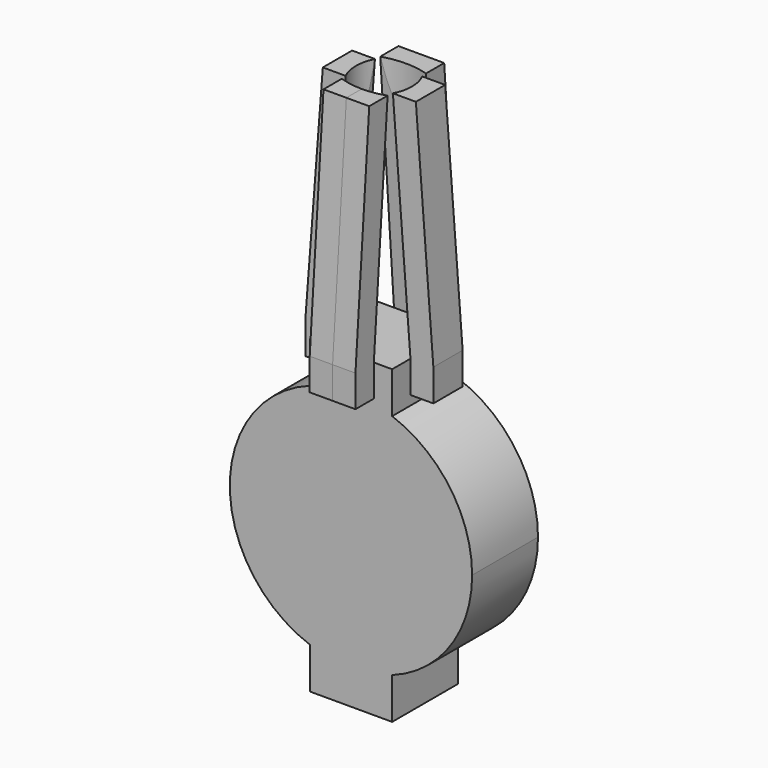
from build123d import *

# Parameters (mm, degrees)
F0_W      = 4.565686686
F0_H      = 1.0178177617
F0_H_2    = 1.0234280489
F0_H_3    = 0.7616141811
F0_H_4    = 0.7546050474
F1_DEPTH  = 4.572
F3_DEPTH  = 1.27
F4_DEPTH  = 1.27
F6_DEPTH  = 3.302
F8_DEPTH  = 1.27
F10_DEPTH = 10.16
F12_DEPTH = 10.16
F14_DEPTH = 10.16
F16_DEPTH = 10.16


with BuildPart() as f1:
    # F0 (on Front) → F1 (new body)
    with BuildSketch(Plane.XZ):
        with BuildLine():
            ThreePointArc((2.2870195098, -6.3278463876), (5.5072772106, -3.865487792), (6.7284543651, 0))
            ThreePointArc((6.7284543651, 0), (5.5072772106, 3.865487792), (2.2870195098, 6.3278463876))
            Line((2.2870195098, 6.3278463876), (2.2870195098, 0))
            Line((2.2870195098, 0), (2.2870195098, -6.3278463876))
        make_face()
        with BuildLine():
            Line((2.2870195098, 0), (2.2870195098, 6.3278463876))
            ThreePointArc((2.2870195098, 6.3278463876), (0.004439497, 6.7284529005), (-2.2786671761, 6.330858871))
            Line((-2.2786671761, 6.330858871), (-2.2786671761, 0))
            Line((-2.2786671761, 0), (0, 0))
            Line((0, 0), (2.2870195098, 0))
        make_face()
        with BuildLine():
            ThreePointArc((-2.2786671761, 6.330858871), (0.004439497, 6.7284529005), (2.2870195098, 6.3278463876))
            Line((2.2870195098, 6.3278463876), (2.2870195098, 6.8423901685))
            Line((2.2870195098, 6.8423901685), (-2.2786671761, 6.8423901685))
            Line((-2.2786671761, 6.8423901685), (-2.2786671761, 6.330858871))
        make_face()
        with BuildLine():
            Line((2.2870195098, -6.8408041261), (2.2870195098, -6.3278463876))
            ThreePointArc((2.2870195098, -6.3278463876), (0.004439497, -6.7284529005), (-2.2786671761, -6.330858871))
            Line((-2.2786671761, -6.330858871), (-2.2786671761, -6.8408041261))
            Line((-2.2786671761, -6.8408041261), (2.2870195098, -6.8408041261))
        make_face()
        with BuildLine():
            ThreePointArc((-2.2786671761, -6.330858871), (0.004439497, -6.7284529005), (2.2870195098, -6.3278463876))
            Line((2.2870195098, -6.3278463876), (2.2870195098, 0))
            Line((2.2870195098, 0), (0, 0))
            Line((0, 0), (-2.2786671761, 0))
            Line((-2.2786671761, 0), (-2.2786671761, -6.330858871))
        make_face()
        with BuildLine():
            Line((-2.2786671761, 0), (-2.2786671761, 6.330858871))
            ThreePointArc((-2.2786671761, 6.330858871), (-6.7284543651, 0), (-2.2786671761, -6.330858871))
            Line((-2.2786671761, -6.330858871), (-2.2786671761, 0))
        make_face()
        with Locations((0.0041761668, 7.3512990493)):
            Rectangle(F0_W, F0_H)
        with Locations((0.0041761668, -7.3525181506)):
            Rectangle(F0_W, F0_H_2)
        with Locations((0.0041761668, 8.2410150208)):
            Rectangle(F0_W, F0_H_3)
        with Locations((0.0041761668, -8.2415346988)):
            Rectangle(F0_W, F0_H_4)
    extrude(amount=F1_DEPTH)

    # F2 (on Right) → F3 (join)
    with BuildSketch(Plane.YZ):
        Polygon((0.3121369207, 8.6214040113), (0, 8.6217308417), (0, 6.8479888141), (1.2692490127, 6.8479888141), (1.2692490127, 8.6204018444), align=None)
        Polygon((-0.9517943535, 21.2794924354), (0, 8.6217308417), (0.3121369207, 8.6214040113), (1.2692490127, 8.6204018444), (0.3121369207, 21.2781690061), align=None)
    extrude(amount=F3_DEPTH)

    # F4 (add): a face of the model
    f4_faces = [f1.faces().sort_by_distance(p)[0] for p in [
        (0, 0.21642848, 14.057832874),
    ]]
    extrude(f4_faces, amount=F4_DEPTH)

    # F5 (on face) → F6 (join)
    with BuildSketch(Plane.XZ.offset(4.572)):
        Polygon((-2.2786671761, 6.8476027809), (-2.2786671761, 8.6218221113), (-2.5794459507, 8.6218221113), (-3.5520868842, 8.6218221113), (-3.5520868842, 6.8476027809), align=None)
        Polygon((-2.5794459507, 8.6218221113), (-2.2786671761, 8.6218221113), (-1.3100903016, 21.2784931064), (-2.5794459507, 21.2784931064), (-3.5520868842, 8.6218221113), align=None)
        Polygon((2.5878376327, 8.6218221113), (2.2870195098, 8.6218221113), (2.2870195098, 6.8476027809), (3.5591647029, 6.8476027809), (3.5591647029, 8.6218221113), align=None)
        Polygon((1.3121798402, 21.2784931064), (2.2870195098, 8.6218221113), (2.5878376327, 8.6218221113), (3.5591647029, 8.6218221113), (2.5878376327, 21.2784931064), align=None)
    extrude(amount=-F6_DEPTH)

    # F7 (on face) → F8 (cut)
    with BuildSketch(Plane.XZ.offset(4.572)):
        Polygon((-2.2786671761, 6.8476027809), (-2.2786671761, 8.6218221113), (-1.3100903016, 21.2784931064), (-2.5794459507, 21.2784931064), (-3.5520868842, 8.6218221113), (-3.5520868842, 6.8476027809), align=None)
        Polygon((1.3121798402, 21.2784931064), (2.2870195098, 8.6218221113), (2.2870195098, 6.8476027809), (3.5591647029, 6.8476027809), (3.5591647029, 8.6218221113), (2.5878376327, 21.2784931064), align=None)
    extrude(amount=-F8_DEPTH, mode=Mode.SUBTRACT)

    # F9 (on face) → F10 (cut)
    with BuildSketch(Plane.XY.offset(21.2784931064)):
        with BuildLine():
            Line((-1.3100903016, -3.302), (-1.3100903016, -1.27))
            ThreePointArc((-1.3100903016, -1.27), (-1.5484129776, -2.286), (-1.3100903016, -3.302))
        make_face()
    extrude(amount=-F10_DEPTH, mode=Mode.SUBTRACT)

    # F11 (on face) → F12 (cut)
    with BuildSketch(Plane(origin=(0, 0.0222801298, 21.2784725075), x_dir=(1, 0, 0), z_dir=(0, 0.0010470732, 0.9999994518))):
        with BuildLine():
            Line((-1.27, -0.9740750174), (1.27, -0.9740750174))
            ThreePointArc((1.27, -0.9740750174), (0, -0.7799036016), (-1.27, -0.9740750174))
        make_face()
    extrude(amount=-F12_DEPTH, mode=Mode.SUBTRACT)

    # F13 (on face) → F14 (cut)
    with BuildSketch(Plane.XY.offset(21.2784931064)):
        with BuildLine():
            Line((1.3121798402, -1.27), (1.3121798402, -3.302))
            ThreePointArc((1.3121798402, -3.302), (1.5627109004, -2.286), (1.3121798402, -1.27))
        make_face()
    extrude(amount=-F14_DEPTH, mode=Mode.SUBTRACT)


with BuildPart() as f3:
    # F2 (on Right) → F3, piece 2 (new body)
    with BuildSketch(Plane.YZ):
        Polygon((-4.5720455237, 6.8546989933), (-4.5720455237, 8.6218202487), (-4.8907813616, 8.6218202487), (-5.8480561711, 8.6218202487), (-5.8480561711, 6.8546989933), align=None)
        Polygon((-4.8907813616, 8.6218202487), (-4.5720455237, 8.6218202487), (-3.6162037868, 21.2794924354), (-4.8907813616, 21.2794924354), (-5.8480561711, 8.6218202487), align=None)
    extrude(amount=F3_DEPTH)


with BuildPart() as f4:
    # F4#2 (new): a face of the model
    f4_2_faces = [f3.part.faces().sort_by_distance(p)[0] for p in [
        (0, -4.790471174, 14.0656200962),
    ]]
    extrude(f4_2_faces, amount=F4_DEPTH)


with BuildPart() as f16_tool:
    # F15 (on face) → F16 (new body)
    with BuildSketch(Plane.XY.offset(21.2794924354)):
        with BuildLine():
            Line((0, -3.6162037868), (0, -3.8295243277))
            ThreePointArc((0, -3.8295243277), (0.6439955035, -3.7758315893), (1.2702000095, -3.6162037868))
            Line((1.2702000095, -3.6162037868), (0, -3.6162037868))
        make_face()
        with BuildLine():
            Line((0, -3.6162037868), (-1.27, -3.6162037868))
            ThreePointArc((-1.27, -3.6162037868), (-0.6438941174, -3.7758150249), (0, -3.8295243277))
            Line((0, -3.8295243277), (0, -3.6162037868))
        make_face()
    extrude(amount=-F16_DEPTH)


with BuildPart() as f3_1:
    add(f3.part)

    # F16: cut by f16_tool
    add(f16_tool.part, mode=Mode.SUBTRACT)


with BuildPart() as f4_1:
    add(f4.part)

    # F16: cut by f16_tool
    add(f16_tool.part, mode=Mode.SUBTRACT)


solid = Compound([f1.part, f3_1.part, f4_1.part])
